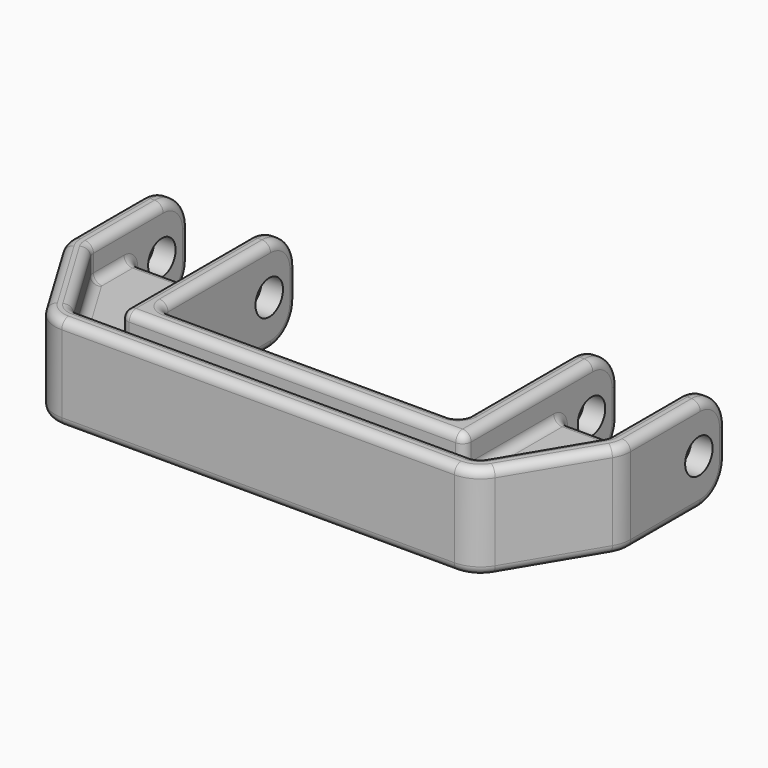
from build123d import *

# Parameters (mm, degrees)
F1_DEPTH  = 22
F2_R      = 7.62
F3_R      = 2.54
F5_R      = 7.62
F6_DEPTH  = 8
F8_DEPTH  = 8
F9_W      = 20
F9_H      = 17
F10_DEPTH = 25.4
F11_F1_R  = 2
F11_F2_R  = 2
F12_R     = 4
F13_DEPTH = 143.002


with BuildPart() as f1:
    # F0 (on Top) → F1 (new body)
    with BuildSketch(Plane.XY):
        Polygon((-35, 30), (-65, 30), (-65, 0), (-50, -25), (0, -25), (0, -10), (-35, -10), align=None)
        Polygon((35, -10), (0, -10), (0, -25), (50, -25), (65, 0), (65, 30), (35, 30), align=None)
    extrude(amount=F1_DEPTH)

    # F2
    f2_edges = [f1.edges().sort_by_distance(p)[0] for p in [
        (50, -25, 11),
        (65, 0, 11),
        (-50, -25, 11),
        (-65, 0, 11),
    ]]
    fillet(f2_edges, radius=F2_R)

    # F3
    f3_edges = [f1.edges().sort_by_distance(p)[0] for p in [
        (35, -10, 11),
        (-35, -10, 11),
    ]]
    fillet(f3_edges, radius=F3_R)

    # F5
    f5_edges = [f1.edges().sort_by_distance(p)[0] for p in [
        (50, 30, 22),
        (50, 30, 0),
        (-50, 30, 22),
        (-50, 30, 0),
    ]]
    fillet(f5_edges, radius=F5_R)

    # F4 (on face) → F6 (cut)
    with BuildSketch(Plane.XY.offset(22)):
        with BuildLine():
            Line((60, 2.1106178129), (60, 25))
            Line((60, 25), (60, 30))
            Line((60, 30), (40, 30))
            Line((40, 30), (40, 25))
            Line((40, 25), (40, -7.46))
            Line((40, -7.46), (40, -15))
            Line((40, -15), (32.46, -15))
            Line((32.46, -15), (-32.46, -15))
            Line((-32.46, -15), (-40, -15))
            Line((-40, -15), (-40, -7.46))
            Line((-40, -7.46), (-40, 25))
            Line((-40, 25), (-40, 30))
            Line((-40, 30), (-60, 30))
            Line((-60, 30), (-60, 25))
            Line((-60, 25), (-60, 2.1106178129))
            ThreePointArc((-60, 2.1106178129), (-59.9049331119, 1.4112518283), (-59.6266314654, 0.7626389337))
            Line((-59.6266314654, 0.7626389337), (-47.9322607776, -18.7279788792))
            ThreePointArc((-47.9322607776, -18.7279788792), (-46.9765002075, -19.6599237557), (-45.6856293123, -20))
            Line((-45.6856293123, -20), (45.6856293123, -20))
            ThreePointArc((45.6856293123, -20), (46.9765002075, -19.6599237557), (47.9322607776, -18.7279788792))
            Line((47.9322607776, -18.7279788792), (59.6266314654, 0.7626389337))
            ThreePointArc((59.6266314654, 0.7626389337), (59.9049331119, 1.4112518283), (60, 2.1106178129))
        make_face()
    extrude(amount=-F6_DEPTH, mode=Mode.SUBTRACT)

    # F7 (on face) → F8 (cut)
    with BuildSketch(Plane(origin=(0, 0, 0), x_dir=(1, 0, 0), z_dir=(0, 0, -1))):
        with BuildLine():
            Line((60, -34.1607518494), (60, -22.38))
            Line((60, -22.38), (60, -2.1106178129))
            ThreePointArc((60, -2.1106178129), (59.9049331119, -1.4112518283), (59.6266314654, -0.7626389337))
            Line((59.6266314654, -0.7626389337), (47.9322607776, 18.7279788792))
            ThreePointArc((47.9322607776, 18.7279788792), (46.9765002075, 19.6599237557), (45.6856293123, 20))
            Line((45.6856293123, 20), (-45.6856293123, 20))
            ThreePointArc((-45.6856293123, 20), (-46.9765002075, 19.6599237557), (-47.9322607776, 18.7279788792))
            Line((-47.9322607776, 18.7279788792), (-59.6266314654, -0.7626389337))
            ThreePointArc((-59.6266314654, -0.7626389337), (-59.9049331119, -1.4112518283), (-60, -2.1106178129))
            Line((-60, -2.1106178129), (-60, -17.38))
            Line((-60, -17.38), (-60, -32.1683958173))
            Line((-60, -32.1683958173), (-40, -32.1683958173))
            Line((-40, -32.1683958173), (-40, -17.38))
            Line((-40, -17.38), (-40, 7.46))
            Line((-40, 7.46), (-40, 15))
            Line((-40, 15), (-32.46, 15))
            Line((-32.46, 15), (32.46, 15))
            Line((32.46, 15), (40, 15))
            Line((40, 15), (40, 7.46))
            Line((40, 7.46), (40, -22.38))
            Line((40, -22.38), (40, -34.1607518494))
            Line((40, -34.1607518494), (60, -34.1607518494))
        make_face()
    extrude(amount=-F8_DEPTH, mode=Mode.SUBTRACT)

    # F9 (on face) → F10 (cut)
    with BuildSketch(Plane(origin=(0, 0, 8), x_dir=(1, 0, 0), z_dir=(0, 0, -1))):
        with Locations((-50, -21.5)):
            Rectangle(F9_W, F9_H)
        with Locations((50, -21.5)):
            Rectangle(F9_W, F9_H)
    extrude(amount=-F10_DEPTH, mode=Mode.SUBTRACT)

    # F11: fillet of radius 2 on 108 edges, made by hand

    # F11_f1
    f11_f1_edges = [f1.edges().sort_by_distance(p)[0] for p in [
        (-60, 12.2453089065, 22),
        (0, -15, 22),
        (-40, 3.69, 22),
        (40, 3.69, 22),
        (40, -15, 18),
        (-40, -15, 18),
        (0, -10, 22),
        (0, -25, 22),
        (50, 13, 14),
        (50, 13, 8),
        (-50, 13, 14),
        (-50, 13, 8),
        (-40, -15, 4),
        (0, -15, 0),
        (40, -15, 4),
        (-35, 7.46, 0),
        (-34.2560512242, -9.2560512242, 0),
        (0, -10, 0),
        (34.2560512242, -9.2560512242, 0),
        (35, 7.46, 0),
        (40, 3.69, 0),
        (-40, 3.69, 0),
        (-40, 27.7681536726, 2.2318463274),
        (-35, 27.7681536726, 2.2318463274),
        (-35, 30, 11),
        (-40, 30, 11),
        (-40, 27.7681536726, 19.7681536726),
        (-35, 27.7681536726, 19.7681536726),
        (-35, 7.46, 22),
        (35, 7.46, 22),
        (34.2560512242, -9.2560512242, 22),
        (-34.2560512242, -9.2560512242, 22),
        (35, 27.7681536726, 19.7681536726),
        (40, 27.7681536726, 19.7681536726),
        (40, 30, 11),
        (35, 30, 11),
        (53.7794461215, -8.9826699728, 22),
        (-65, 12.2453089065, 22),
        (-64.723507753, 0.0765839189, 22),
        (-58.0669107501, -11.5551487499, 22),
        (-49.4399942824, -24.0109232895, 22),
        (49.4399942824, -24.0109232895, 22),
        (58.0669107501, -11.5551487499, 22),
        (64.723507753, 0.0765839189, 22),
        (65, 12.2453089065, 22),
        (60, 12.2453089065, 22),
        (59.9049331119, 1.4112518283, 22),
        (46.9765002075, -19.6599237557, 22),
        (0, -20, 22),
        (-46.9765002075, -19.6599237557, 22),
        (-53.7794461215, -8.9826699728, 22),
        (-59.9049331119, 1.4112518283, 22),
        (60, 27.7681536726, 19.7681536726),
        (65, 27.7681536726, 19.7681536726),
        (65, 30, 11),
        (60, 30, 11),
        (60, 27.7681536726, 2.2318463274),
        (65, 27.7681536726, 2.2318463274),
        (-60, 12.2453089065, 0),
        (-59.9049331119, 1.4112518283, 0),
        (-53.7794461215, -8.9826699728, 0),
        (-46.9765002075, -19.6599237557, 0),
        (0, -20, 0),
        (46.9765002075, -19.6599237557, 0),
        (53.7794461215, -8.9826699728, 0),
        (59.9049331119, 1.4112518283, 0),
        (60, 12.2453089065, 0),
        (65, 12.2453089065, 0),
        (64.723507753, 0.0765839189, 0),
        (58.0669107501, -11.5551487499, 0),
        (49.4399942824, -24.0109232895, 0),
        (0, -25, 0),
        (-49.4399942824, -24.0109232895, 0),
        (-58.0669107501, -11.5551487499, 0),
        (-64.723507753, 0.0765839189, 0),
        (-65, 12.2453089065, 0),
        (-65, 27.7681536726, 2.2318463274),
        (-60, 27.7681536726, 2.2318463274),
        (-60, 30, 11),
        (-65, 30, 11),
        (-65, 27.7681536726, 19.7681536726),
        (-60, 27.7681536726, 19.7681536726),
        (40, 27.7681536726, 2.2318463274),
        (35, 27.7681536726, 2.2318463274),
    ]]
    fillet(f11_f1_edges, radius=F11_F1_R)

    # F11_f2
    f11_f2_edges = [f1.edges().sort_by_distance(p)[0] for p in [
        (0, -20, 14),
        (-40, -1, 14),
        (0, -15, 14),
        (46.9765002075, -19.6599237557, 14),
        (-46.9765002075, -19.6599237557, 14),
        (-53.7794461215, -8.9826699728, 14),
        (-59.9049331119, 1.4112518283, 14),
        (-60, 6.5553089065, 14),
        (40, -1, 14),
        (60, 6.5553089065, 14),
        (59.9049331119, 1.4112518283, 14),
        (53.7794461215, -8.9826699728, 14),
        (59.9049331119, 1.4112518283, 8),
        (40, -1, 8),
        (0, -15, 8),
        (-40, -1, 8),
        (-60, 6.5553089065, 8),
        (-59.9049331119, 1.4112518283, 8),
        (-53.7794461215, -8.9826699728, 8),
        (-46.9765002075, -19.6599237557, 8),
        (0, -20, 8),
        (46.9765002075, -19.6599237557, 8),
        (53.7794461215, -8.9826699728, 8),
        (60, 6.5553089065, 8),
        (60, 12.4142135624, 8.5857864376),
        (-60, 12.4142135624, 8.5857864376),
        (-40, 12.4142135624, 8.5857864376),
        (-39.4142135624, -14.4142135624, 8),
        (39.4142135624, -14.4142135624, 8),
        (40, 12.4142135624, 8.5857864376),
        (60, 12.4142135624, 13.4142135624),
        (40, 12.4142135624, 13.4142135624),
        (39.4142135624, -14.4142135624, 14),
        (-60, 12.4142135624, 13.4142135624),
        (-39.4142135624, -14.4142135624, 14),
        (-40, 12.4142135624, 13.4142135624),
    ]]
    fillet(f11_f2_edges, radius=F11_F2_R)

    # F12 (on face) → F13 (cut)
    with BuildSketch(Plane.YZ.offset(65)):
        with Locations((22, 11)):
            Circle(F12_R)
    extrude(amount=-F13_DEPTH, mode=Mode.SUBTRACT)


solid = f1.part
